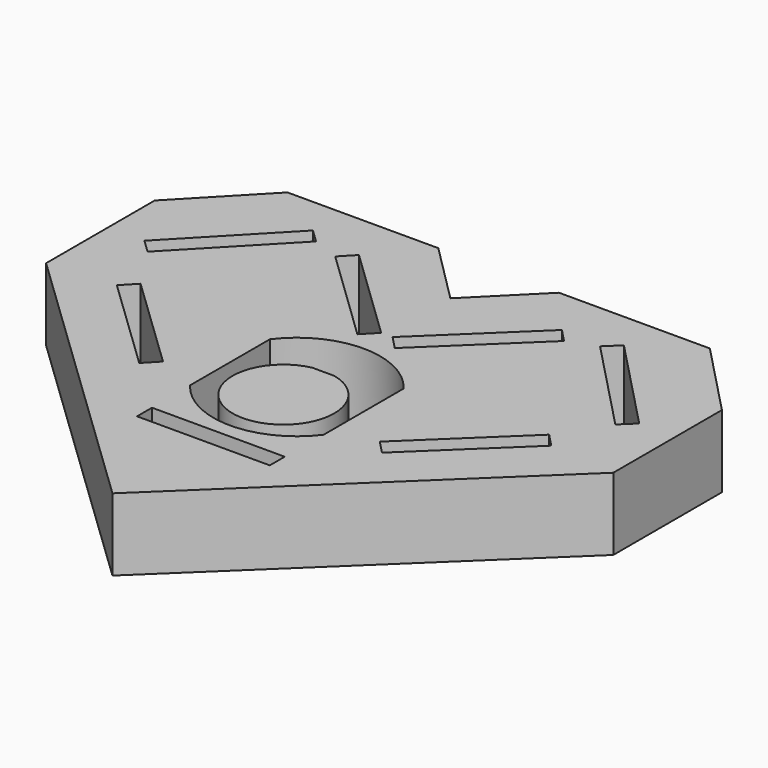
from build123d import *

# Parameters (mm, degrees)
F1_DEPTH = 12
F2_W     = 22
F2_H     = 3.1
F3_DEPTH = 25


# Not quite as in the source:
# - a feature names something its author has since deleted; it is built from what else it names


with BuildPart() as f1:
    # F0 (on Top) → F1 (new body)
    with BuildSketch(Plane.XY):
        Polygon((-47, -16), (0, -61), (47, -16), (47, 6.5), (35, 19), (10, 19), (0, 9), (-10, 19), (-35, 19), (-47, 6.5), align=None)
    extrude(amount=F1_DEPTH)

    # F2 (on face) → F3 (cut)
    with BuildSketch(Plane.XY.offset(12)):
        Polygon((38.7636993048, -5.2805951643), (41, -3.1337464969), (25.7642997798, 12.7367745658), (23.5279990846, 10.5899258984), align=None)
        Polygon((17.9653521283, -28.0733723465), (20.1092237756, -30.3125271781), (36, -15.0979541973), (33.8561283527, -12.8587993657), align=None)
        with Locations((0, -40.611379497)):
            Rectangle(F2_W, F2_H)
        Polygon((-17.9653521283, -28.0733723465), (-33.8561283527, -12.8587993657), (-36, -15.0979541973), (-20.1092237756, -30.3125271781), align=None)
        Polygon((3.0954246037, -6.3915316387), (18.9659456664, 8.8441685815), (16.819096999, 11.0804692767), (0.9485759364, -4.1552309435), align=None)
        Polygon((-18.9659456664, 8.8441685815), (-3.0954246037, -6.3915316387), (-0.9485759364, -4.1552309435), (-16.819096999, 11.0804692767), align=None)
        Polygon((-38.7636993048, -5.2805951643), (-23.5279990846, 10.5899258984), (-25.7642997798, 12.7367745658), (-41, -3.1337464969), align=None)
        with BuildLine():
            Line((-11.0683567197, -14.5500370711), (-11.0683567197, -31.0999615422))
            ThreePointArc((-11.0683567197, -31.0999615422), (0.0066432803, -36.6499993066), (11.0816432803, -31.0999615422))
            Line((11.0816432803, -31.0999615422), (11.0816432803, -14.5500370711))
            ThreePointArc((11.0816432803, -14.5500370711), (0.0066432803, -8.9999993066), (-11.0683567197, -14.5500370711))
        make_face()
        with BuildLine():
            ThreePointArc((1.8566432803, -17.3596185624), (-0.0296329992, -33.9999209479), (-1.8433567197, -17.3515544229))
            Line((-1.8433567197, -17.3515544229), (1.8566432803, -17.3596185624))
        make_face(mode=Mode.SUBTRACT)
    extrude(amount=-F3_DEPTH, mode=Mode.SUBTRACT)


solid = f1.part
